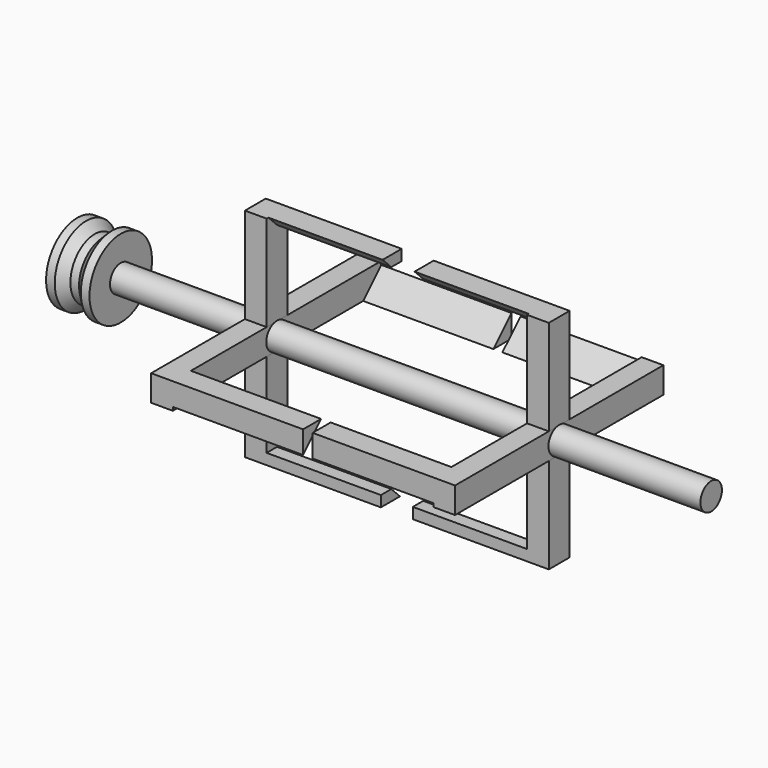
from build123d import *

# Parameters (mm, degrees)
F0_W           = 175
F0_H           = 15.5
F0_W_2         = 25
F2_DEPTH       = 15
F4_DEPTH       = 15
F5_T1_DEPTH    = 150
F5_2_T1_DEPTH  = 139.6191499531
F5_2_T3_DEPTH  = 139.0574328601
F6_R           = 50
F7_DEPTH       = 20
F8_R           = 45
F9_DEPTH       = 20
F10_R          = 35
F11_DEPTH      = 10
F12_R          = 45
F13_DEPTH      = 20
F14_SIZE       = 9.99999
F15_T1_DEPTH   = 170.1724504435
F15_2_T1_DEPTH = 170.1724504435
F16_T1_DEPTH   = 170.1724504435
F16_2_T1_DEPTH = 170.1724504435
F0_W_3         = 300


# Not quite as in the source:
# - a fillet or chamfer that OpenCascade refuses, or shapes differently, is made with other operations: its cross-section is extruded or revolved along the edge and cut away or added
# - a fillet or chamfer is up to 0.001 mm smaller than in the source, because OpenCascade refuses the exact size
# - a feature names something its author has since deleted; it is built from what else it names


with BuildPart() as f1:
    # F0 (on Front) → F1 (revolve)
    with BuildSketch(Plane.XZ):
        with Locations((262.5, 7.75)):
            Rectangle(F0_W, F0_H)
    revolve(axis=Axis((0, 0, 0), (-1, 0, 0)))


with BuildPart() as f1b:
    # F0 (on Front) → F1, piece 2 (revolve)
    with BuildSketch(Plane.XZ):
        with Locations((-262.5, 7.75)):
            Rectangle(F0_W, F0_H)
    revolve(axis=Axis((0, 0, 0), (-1, 0, 0)))

    # F6 (on face) → F7 (cut)
    with BuildSketch(Plane(origin=(-350, 0, 0), x_dir=(0, -1, 0), z_dir=(-1, 0, 0))):
        Circle(F6_R)
    extrude(amount=-F7_DEPTH, mode=Mode.SUBTRACT)

    # F8 (on face) → F9 (join)
    with BuildSketch(Plane(origin=(-330, 0, 0), x_dir=(0, -1, 0), z_dir=(-1, 0, 0))):
        Circle(F8_R)
    extrude(amount=F9_DEPTH)

    # F10 (on face) → F11 (join)
    with BuildSketch(Plane(origin=(-350, 0, 0), x_dir=(0, -1, 0), z_dir=(-1, 0, 0))):
        Circle(F10_R)
    extrude(amount=F11_DEPTH)

    # F12 (on face) → F13 (join)
    with BuildSketch(Plane(origin=(-360, 0, 0), x_dir=(0, -1, 0), z_dir=(-1, 0, 0))):
        Circle(F12_R)
    extrude(amount=F13_DEPTH)

    # F14 (size 10 in the source; OpenCascade refuses exactly that, so slightly less here)
    f14_edges = [f1b.edges().sort_by_distance(p)[0] for p in [
        (-350, 45, 0),
        (-360, 45, 0),
    ]]
    chamfer(f14_edges, length=F14_SIZE)


with BuildPart() as f2:
    # F0 (on Front) → F2 (new body, symmetric)
    with BuildSketch(Plane.XZ):
        Polygon((-150, -15.5), (-175, -15.5), (-175, -125), (-18.402794376, -125), (-18.402794376, -112.5), (-150, -112.5), align=None)
        Polygon((-175, 125), (-175, 15.5), (-150, 15.5), (-150, 112.5), (-18.402794376, 112.5), (-18.402794376, 125), align=None)
        with Locations((-162.5, 7.75)):
            Rectangle(F0_W_2, F0_H)
        with Locations((-162.5, -7.75)):
            Rectangle(F0_W_2, F0_H)
    extrude(amount=F2_DEPTH, both=True)

    # F15: chamfer of 15 on 1 edges, made by hand

    # F15_s2 → F15_t1 (cut)
    with BuildSketch(Plane.YZ.offset(-150)):
        Polygon((0, 112.5), (-15, 127.5), (-15, 112.5), align=None)
    extrude(amount=F15_T1_DEPTH, mode=Mode.SUBTRACT)

    # F16: chamfer of 15 on 1 edges, made by hand

    # F16_s2 → F16_t1 (cut)
    with BuildSketch(Plane.YZ.offset(-150)):
        Polygon((0, -112.5), (15, -127.5), (15, -112.5), align=None)
    extrude(amount=F16_T1_DEPTH, mode=Mode.SUBTRACT)


with BuildPart() as f2b:
    # F0 (on Front) → F2, piece 2 (new body, symmetric)
    with BuildSketch(Plane.XZ):
        Polygon((175, -15.5), (150, -15.5), (150, -112.5), (18.402794376, -112.5), (18.402794376, -125), (175, -125), align=None)
        Polygon((150, 112.5), (150, 15.5), (175, 15.5), (175, 125), (18.402794376, 125), (18.402794376, 112.5), align=None)
        with Locations((162.5, 7.75)):
            Rectangle(F0_W_2, F0_H)
        with Locations((162.5, -7.75)):
            Rectangle(F0_W_2, F0_H)
    extrude(amount=F2_DEPTH, both=True)

    # F15#2: chamfer of 15 on 1 edges, made by hand

    # F15_2_s2 → F15_2_t1 (cut)
    with BuildSketch(Plane.YZ.offset(-20.1724504435)):
        Polygon((0, 112.5), (-15, 127.5), (-15, 112.5), align=None)
    extrude(amount=F15_2_T1_DEPTH, mode=Mode.SUBTRACT)

    # F16#2: chamfer of 15 on 1 edges, made by hand

    # F16_2_s2 → F16_2_t1 (cut)
    with BuildSketch(Plane.YZ.offset(-20.1724504435)):
        Polygon((0, -112.5), (15, -127.5), (15, -112.5), align=None)
    extrude(amount=F16_2_T1_DEPTH, mode=Mode.SUBTRACT)


with BuildPart() as f4:
    # F3 (on Top) → F4 (new body, symmetric)
    with BuildSketch(Plane.XY):
        Polygon((175, -150), (175, 150), (10.3808500469, 150), (10.3808500469, 124), (150, 124), (150, -124), (10.9425671399, -124), (10.9425671399, -150), align=None)
    extrude(amount=F4_DEPTH, both=True)

    # F5#2: chamfer of 30 on 2 edges, made by hand

    # F5_2_s2 → F5_2_t1 (cut)
    with BuildSketch(Plane.YZ.offset(10.3808500469)):
        with BuildLine():
            Line((123.1514718626, -15.8485281374), (154.8485281374, 15.8485281374))
            Line((154.8485281374, 15.8485281374), (154.8485281374, 16.4485281374))
            ThreePointArc((154.8485281374, 16.4485281374), (139.4242640687, 15.6), (124, 15.6))
            Line((124, 15.6), (123.4, 15))
            ThreePointArc((123.4, 15), (123.4, -0.4242640687), (122.5514718626, -15.8485281374))
            Line((122.5514718626, -15.8485281374), (123.1514718626, -15.8485281374))
        make_face()
    extrude(amount=F5_2_T1_DEPTH, mode=Mode.SUBTRACT)

    # F5_2_s4 → F5_2_t3 (cut)
    with BuildSketch(Plane.YZ.offset(10.9425671399)):
        with BuildLine():
            Line((-123.1514718626, 15.8485281374), (-154.8485281374, -15.8485281374))
            Line((-154.8485281374, -15.8485281374), (-154.8485281374, -16.4485281374))
            ThreePointArc((-154.8485281374, -16.4485281374), (-139.4242640687, -15.6), (-124, -15.6))
            Line((-124, -15.6), (-123.4, -15))
            ThreePointArc((-123.4, -15), (-123.4, 0.4242640687), (-122.5514718626, 15.8485281374))
            Line((-122.5514718626, 15.8485281374), (-123.1514718626, 15.8485281374))
        make_face()
    extrude(amount=F5_2_T3_DEPTH, mode=Mode.SUBTRACT)


with BuildPart() as f4b:
    # F3 (on Top) → F4, piece 2 (new body, symmetric)
    with BuildSketch(Plane.XY):
        Polygon((0, 150), (-175, 150), (-175, -150), (0, -150), (0, -124), (-150, -124), (-150, 124), (0, 124), align=None)
    extrude(amount=F4_DEPTH, both=True)

    # F5: chamfer of 30 on 2 edges, made by hand

    # F5_s2 → F5_t1 (cut)
    with BuildSketch(Plane.YZ.offset(-150)):
        with BuildLine():
            Line((123.1514718626, -15.8485281374), (154.8485281374, 15.8485281374))
            Line((154.8485281374, 15.8485281374), (154.8485281374, 16.4485281374))
            ThreePointArc((154.8485281374, 16.4485281374), (139.4242640687, 15.6), (124, 15.6))
            Line((124, 15.6), (123.4, 15))
            ThreePointArc((123.4, 15), (123.4, -0.4242640687), (122.5514718626, -15.8485281374))
            Line((122.5514718626, -15.8485281374), (123.1514718626, -15.8485281374))
        make_face()
        with BuildLine():
            Line((-123.1514718626, 15.8485281374), (-154.8485281374, -15.8485281374))
            Line((-154.8485281374, -15.8485281374), (-154.8485281374, -16.4485281374))
            ThreePointArc((-154.8485281374, -16.4485281374), (-139.4242640687, -15.6), (-124, -15.6))
            Line((-124, -15.6), (-123.4, -15))
            ThreePointArc((-123.4, -15), (-123.4, 0.4242640687), (-122.5514718626, 15.8485281374))
            Line((-122.5514718626, 15.8485281374), (-123.1514718626, 15.8485281374))
        make_face()
    extrude(amount=F5_T1_DEPTH, mode=Mode.SUBTRACT)


with BuildPart() as f17:
    # F0 (on Front) → F17 (revolve)
    with BuildSketch(Plane.XZ):
        with Locations((0, -7.75)):
            Rectangle(F0_W_3, F0_H)
    revolve(axis=Axis((0, 0, 0), (-1, 0, 0)))


solid = Compound([f1.part, f1b.part, f2.part, f2b.part, f4.part, f4b.part, f17.part])
